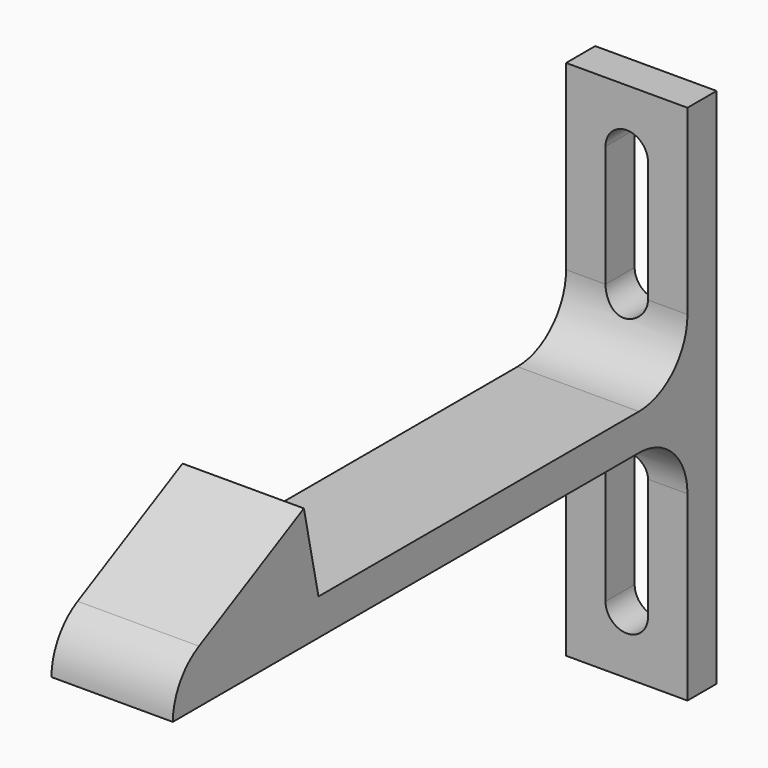
from build123d import *

# Parameters (mm, degrees)
F1_DEPTH    = 5
F3_DEPTH    = 3.001
F5_DEPTH    = 25
F6_T4_DEPTH = 10
F6_S5_R     = 1.75
F6_T6_DEPTH = 8
F7_T4_DEPTH = 10
F7_S5_R     = 1.75
F7_T6_DEPTH = 8
F8_T1_DEPTH = 25.1979746773


# Not quite as in the source:
# - a fillet or chamfer that OpenCascade refuses, or shapes differently, is made with other operations: its cross-section is extruded or revolved along the edge and cut away or added


with BuildPart() as f1:
    # F0 (on Right) → F1 (new body, symmetric)
    with BuildSketch(Plane.YZ):
        Polygon((0, 20), (0, 0), (-38, 0), (-39.5, 7), (-53, 0), (-53, -3), (0, -3), (0, -23), (3, -23), (3, 20), align=None)
    extrude(amount=F1_DEPTH, both=True)

    # F2 (on face) → F3 (cut, through all)
    with BuildSketch(Plane.XZ):
        with BuildLine():
            ThreePointArc((-1.75, 15), (0, 13.25), (1.75, 15))
            ThreePointArc((1.75, 15), (0, 16.75), (-1.75, 15))
        make_face()
        with BuildLine():
            Line((1.75, 5), (1.75, 15))
            ThreePointArc((1.75, 15), (0, 13.25), (-1.75, 15))
            Line((-1.75, 15), (-1.75, 5))
            ThreePointArc((-1.75, 5), (0, 6.75), (1.75, 5))
        make_face()
        with BuildLine():
            Line((0, 5), (1.75, 5))
            ThreePointArc((1.75, 5), (0, 6.75), (-1.75, 5))
            Line((-1.75, 5), (0, 5))
        make_face()
        with BuildLine():
            ThreePointArc((-1.75, 5), (0, 3.25), (1.75, 5))
            Line((1.75, 5), (0, 5))
            Line((0, 5), (-1.75, 5))
        make_face()
    extrude(amount=-F3_DEPTH, mode=Mode.SUBTRACT)

    # F4 (on face) → F5 (cut)
    with BuildSketch(Plane.XZ):
        with BuildLine():
            ThreePointArc((-1.75, -18), (0, -19.75), (1.75, -18))
            ThreePointArc((1.75, -18), (0, -16.25), (-1.75, -18))
        make_face()
        with BuildLine():
            Line((1.75, -18), (1.75, -8))
            ThreePointArc((1.75, -8), (0, -9.75), (-1.75, -8))
            Line((-1.75, -8), (-1.75, -18))
            ThreePointArc((-1.75, -18), (0, -16.25), (1.75, -18))
        make_face()
        with BuildLine():
            ThreePointArc((-1.75, -8), (0, -9.75), (1.75, -8))
            ThreePointArc((1.75, -8), (0, -6.25), (-1.75, -8))
        make_face()
    extrude(amount=-F5_DEPTH, mode=Mode.SUBTRACT)

    # F6: fillet of radius 5 on 1 edges, made by hand


with BuildPart() as f6_tool2:
    # F6_s3 → F6_t4 (new body)
    with BuildSketch(Plane.YZ.offset(-5)):
        with BuildLine():
            ThreePointArc((0, 5), (-1.4644660941, 1.4644660941), (-5, 0))
            Line((-5, 0), (0, 0))
            Line((0, 0), (0, 5))
        make_face()
    extrude(amount=F6_T4_DEPTH)

    # F6_s5 → F6_t6 (cut, symmetric)
    with BuildSketch(Plane.XZ.offset(2.5)):
        with Locations((0, 5)):
            Circle(F6_S5_R)
    extrude(amount=F6_T6_DEPTH, both=True, mode=Mode.SUBTRACT)


with BuildPart() as f1_1:
    add(f1.part)

    # F6_t1: union F6_tool2
    add(f6_tool2.part)

    # F7: fillet of radius 5 on 1 edges, made by hand


with BuildPart() as f7_tool2:
    # F7_s3 → F7_t4 (new body)
    with BuildSketch(Plane.YZ.offset(-5)):
        with BuildLine():
            ThreePointArc((-5, -3), (-1.4644660941, -4.4644660941), (0, -8))
            Line((0, -8), (0, -3))
            Line((0, -3), (-5, -3))
        make_face()
    extrude(amount=F7_T4_DEPTH)

    # F7_s5 → F7_t6 (cut, symmetric)
    with BuildSketch(Plane.XZ.offset(2.5)):
        with Locations((0, -8)):
            Circle(F7_S5_R)
    extrude(amount=F7_T6_DEPTH, both=True, mode=Mode.SUBTRACT)


with BuildPart() as f1_2:
    add(f1_1.part)

    # F7_t1: union F7_tool2
    add(f7_tool2.part)

    # F8: fillet of radius 5 on 1 edges, made by hand

    # F8_s2 → F8_t1 (cut)
    with BuildSketch(Plane.YZ.offset(-12.5989873387)):
        with BuildLine():
            ThreePointArc((-50.3015858223, 1.3991777218), (-52.2724658636, -0.4422818153), (-53, -3.0395949355))
            Line((-53, -3.0395949355), (-53, 0))
            Line((-53, 0), (-50.3015858223, 1.3991777218))
        make_face()
    extrude(amount=F8_T1_DEPTH, mode=Mode.SUBTRACT)


solid = f1_2.part
